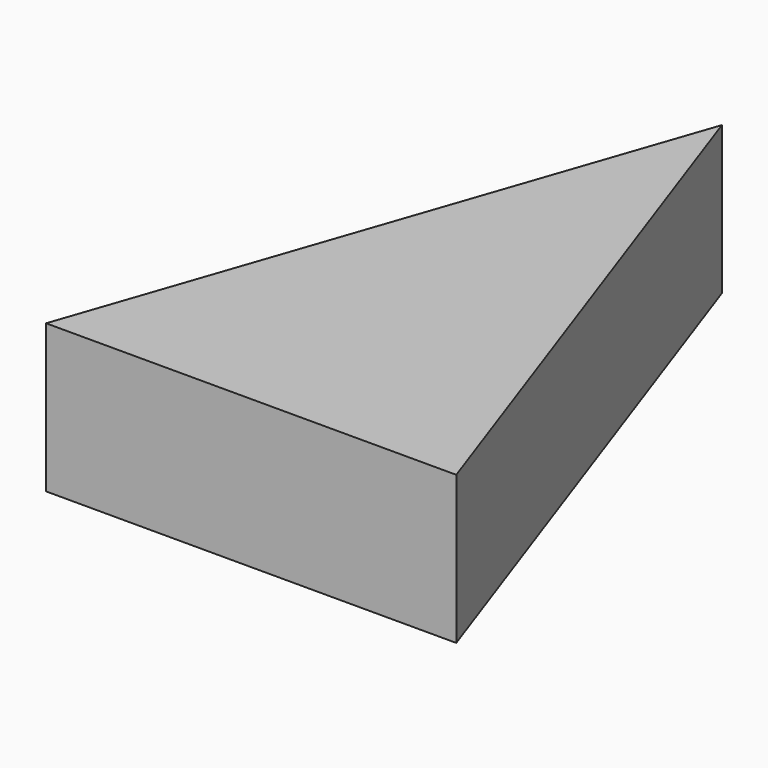
from build123d import *

# Parameters (mm, degrees)
F1_DEPTH = 6.35


# Not quite as in the source:
# - a feature of the source that left no trace in its solid (it failed there, or was rolled back) is left out


with BuildPart() as f1:
    # F0 (on Top) → F1 (new body)
    with BuildSketch(Plane.XY):
        Polygon((-8.6967386305, 0), (0, 0), (0, 25.3740157932), align=None)
        Polygon((0, 25.3740157932), (0, 0), (8.9013688266, 0), align=None)
    extrude(amount=F1_DEPTH)


solid = f1.part
